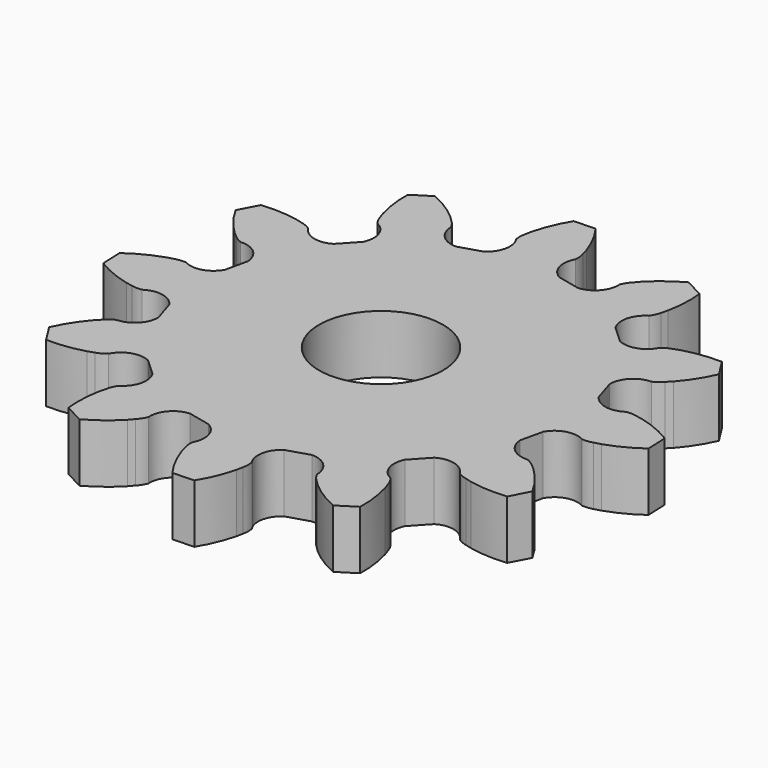
from build123d import *

# Parameters (mm, degrees)
F0_R     = 3.175
F1_DEPTH = 6
F2_R     = 6.35
F3_DEPTH = 6


# Not quite as in the source:
# - ends of sketch curves that miss each other by under 0.0002 mm in the source are joined


with BuildPart() as f1:
    # F0 (on Top) → F1 (new body)
    with BuildSketch(Plane.XY):
        with BuildLine():
            ThreePointArc((8.0856551802, 20.4586539905), (7.495744634, 18.7245439088), (5.8524138883, 17.9154726581))
            Line((5.8524138883, 17.9154726581), (3.533593868, 18.4377149703))
            ThreePointArc((3.533593868, 18.4377149703), (2.39577008, 19.8731553984), (2.6062168473, 21.6927279818))
            ThreePointArc((2.6062168473, 21.6927279818), (2.5956181006, 22.2379348343), (2.4812105153, 22.7711081757))
            Line((2.4812105153, 22.7711081757), (2.304819868, 23.4221699703))
            ThreePointArc((2.304819868, 23.4221699703), (1.5537928627, 25.1976657599), (0.5382999658, 26.8363240419))
            Line((0.5382999658, 26.8363240419), (-1.652266132, 26.7480479703))
            ThreePointArc((-1.652266132, 26.7480479703), (-2.5326105159, 25.0329912972), (-3.1383352523, 23.202821))
            Line((-3.1383352523, 23.202821), (-3.261765132, 22.5396759703))
            ThreePointArc((-3.261765132, 22.5396759703), (-3.3328999602, 21.9990293129), (-3.299595445, 21.4547409207))
            ThreePointArc((-3.299595445, 21.4547409207), (-2.9434159043, 19.6579951944), (-3.962046635, 18.1356532254))
            Line((-3.962046635, 18.1356532254), (-6.231325132, 17.4285189703))
            ThreePointArc((-6.231325132, 17.4285189703), (-7.9344291384, 18.1027349909), (-8.6619631428, 19.7837539701))
            ThreePointArc((-8.6619631428, 19.7837539701), (-8.9437456025, 20.2506173173), (-9.3094119635, 20.6551551548))
            Line((-9.3094119635, 20.6551551548), (-9.787702132, 21.1307969703))
            ThreePointArc((-9.787702132, 21.1307969703), (-11.3258583806, 22.2929078915), (-13.0246300842, 23.2042810788))
            Line((-13.0246300842, 23.2042810788), (-14.877578132, 22.0325489703))
            ThreePointArc((-14.877578132, 22.0325489703), (-14.7824500692, 20.1070937471), (-14.3919378876, 18.2192570409))
            Line((-14.3919378876, 18.2192570409), (-14.167259132, 17.5832419703))
            ThreePointArc((-14.167259132, 17.5832419703), (-13.9585396302, 17.0794612267), (-13.6575531356, 16.6247459674))
            ThreePointArc((-13.6575531356, 16.6247459674), (-12.450720223, 15.2468077423), (-12.5717095188, 13.4191061613))
            Line((-12.5717095188, 13.4191061613), (-14.183394132, 11.6720709703))
            ThreePointArc((-14.183394132, 11.6720709703), (-15.9954339265, 11.4044064302), (-17.4660067474, 12.4964452005))
            ThreePointArc((-17.4660067474, 12.4964452005), (-17.9434693275, 12.7598688849), (-18.4624142066, 12.9273756305))
            Line((-18.4624142066, 12.9273756305), (-19.114446132, 13.1001489703))
            ThreePointArc((-19.114446132, 13.1001489703), (-21.0275840666, 13.3374876551), (-22.954450043, 13.2773741537))
            Line((-22.954450043, 13.2773741537), (-23.973284132, 11.3361509703))
            ThreePointArc((-23.973284132, 11.3361509703), (-22.9281735093, 9.7162222135), (-21.646062089, 8.276564015))
            Line((-21.646062089, 8.276564015), (-21.133476132, 7.8380979703))
            ThreePointArc((-21.133476132, 7.8380979703), (-20.700829784, 7.5061704221), (-20.2128101981, 7.2628687982))
            ThreePointArc((-20.2128101981, 7.2628687982), (-18.4786930704, 6.6729557362), (-17.6696218198, 5.0296249905))
            Line((-17.6696218198, 5.0296249905), (-18.191865132, 2.7108049703))
            ThreePointArc((-18.191865132, 2.7108049703), (-19.6273047939, 1.5729811157), (-21.4468771435, 1.7834279496))
            ThreePointArc((-21.4468771435, 1.7834279496), (-21.992083996, 1.7728292029), (-22.5252573374, 1.6584216176))
            Line((-22.5252573374, 1.6584216176), (-23.176320132, 1.4820309703))
            ThreePointArc((-23.176320132, 1.4820309703), (-24.951815701, 0.7310035617), (-26.5904738545, -0.2844894086))
            Line((-26.5904738545, -0.2844894086), (-26.502198132, -2.4750550297))
            ThreePointArc((-26.502198132, -2.4750550297), (-24.7871404994, -3.3553983967), (-22.9569699288, -3.9611232076))
            Line((-22.9569699288, -3.9611232076), (-22.293825132, -4.0845540297))
            ThreePointArc((-22.293825132, -4.0845540297), (-21.7531784746, -4.1556888579), (-21.2088900824, -4.1223843427))
            ThreePointArc((-21.2088900824, -4.1223843427), (-19.4121448118, -3.7662049106), (-17.8898035408, -4.7848353025))
            Line((-17.8898035408, -4.7848353025), (-17.182669132, -7.0541130297))
            ThreePointArc((-17.182669132, -7.0541130297), (-17.8568848047, -8.7572176771), (-19.5379041318, -9.4847520406))
            ThreePointArc((-19.5379041318, -9.4847520406), (-20.0047679489, -9.7665338494), (-20.4093058145, -10.1322004067))
            Line((-20.4093058145, -10.1322004067), (-20.884947132, -10.6104910297))
            ThreePointArc((-20.884947132, -10.6104910297), (-22.0470577895, -12.1486474277), (-22.9584307722, -13.8474191883))
            Line((-22.9584307722, -13.8474191883), (-21.786699132, -15.7003670297))
            ThreePointArc((-21.786699132, -15.7003670297), (-19.8612438949, -15.6052379651), (-17.9734072026, -15.2147257853))
            Line((-17.9734072026, -15.2147257853), (-17.337391132, -14.9900470297))
            ThreePointArc((-17.337391132, -14.9900470297), (-16.8336102162, -14.7813279046), (-16.3788950361, -14.4803411482))
            ThreePointArc((-16.3788950361, -14.4803411482), (-15.0009577532, -13.2735084084), (-13.1732557298, -13.3944972155))
            Line((-13.1732557298, -13.3944972155), (-11.426220132, -15.0061830297))
            ThreePointArc((-11.426220132, -15.0061830297), (-11.1585555293, -16.8182225752), (-12.2505939215, -18.2887953813))
            ThreePointArc((-12.2505939215, -18.2887953813), (-12.5140190857, -18.7662573158), (-12.6815259557, -19.2852028487))
            Line((-12.6815259557, -19.2852028487), (-12.854298132, -19.9372350297))
            ThreePointArc((-12.854298132, -19.9372350297), (-13.0916378147, -21.8503729188), (-13.0315243037, -23.7772390484))
            Line((-13.0315243037, -23.7772390484), (-11.090300132, -24.7960730297))
            ThreePointArc((-11.090300132, -24.7960730297), (-9.4703714624, -23.7509617127), (-8.0307131966, -22.4688499676))
            Line((-8.0307131966, -22.4688499676), (-7.592247132, -21.9562650297))
            ThreePointArc((-7.592247132, -21.9562650297), (-7.2603195838, -21.5236186817), (-7.0170179599, -21.0355990958))
            ThreePointArc((-7.0170179599, -21.0355990958), (-6.4271048979, -19.3014819682), (-4.7837741522, -18.4924107175))
            Line((-4.7837741522, -18.4924107175), (-2.464955132, -19.0146530297))
            ThreePointArc((-2.464955132, -19.0146530297), (-1.3271304637, -20.4500930376), (-1.5375771112, -22.2696660413))
            ThreePointArc((-1.5375771112, -22.2696660413), (-1.526978382, -22.8148727434), (-1.4125708708, -23.3480459468))
            Line((-1.4125708708, -23.3480459468), (-1.236180132, -23.9991090297))
            ThreePointArc((-1.236180132, -23.9991090297), (-0.4851536505, -25.7746047396), (0.5303392469, -27.4132627523))
            Line((0.5303392469, -27.4132627523), (2.720904868, -27.3249870297))
            ThreePointArc((2.720904868, -27.3249870297), (3.6012490873, -25.6099297494), (4.2069739883, -23.7797590594))
            Line((4.2069739883, -23.7797590594), (4.330403868, -23.1166140297))
            ThreePointArc((4.330403868, -23.1166140297), (4.4015386962, -22.5759673723), (4.368234181, -22.0316789801))
            ThreePointArc((4.368234181, -22.0316789801), (4.012054776, -20.2349335738), (5.0306858327, -18.7125919768))
            Line((5.0306858327, -18.7125919768), (7.299963868, -18.0054580297))
            ThreePointArc((7.299963868, -18.0054580297), (9.003068504, -18.6796726914), (9.7306028786, -20.3606920138))
            ThreePointArc((9.7306028786, -20.3606920138), (10.0123843385, -20.8275553767), (10.3780506996, -21.2320932142))
            Line((10.3780506996, -21.2320932142), (10.856340868, -21.7077350297))
            ThreePointArc((10.856340868, -21.7077350297), (12.3944972864, -22.8698460597), (14.0932691892, -23.7812193009))
            Line((14.0932691892, -23.7812193009), (15.946216868, -22.6094870297))
            ThreePointArc((15.946216868, -22.6094870297), (15.8510888659, -20.684032283), (15.4605768903, -18.7961960233))
            Line((15.4605768903, -18.7961960233), (15.235897868, -18.1601800297))
            ThreePointArc((15.235897868, -18.1601800297), (15.0271791498, -17.6563988792), (14.7261924755, -17.2016835377))
            ThreePointArc((14.7261924755, -17.2016835377), (13.5193592467, -15.8237466509), (13.6403480539, -13.9960446276))
            Line((13.6403480539, -13.9960446276), (15.252033868, -12.2490090297))
            ThreePointArc((15.252033868, -12.2490090297), (17.0640734135, -11.981344427), (18.5346462196, -13.0733828192))
            ThreePointArc((18.5346462196, -13.0733828192), (19.0121081541, -13.3368079834), (19.531053687, -13.5043148535))
            Line((19.531053687, -13.5043148535), (20.183085868, -13.6770870297))
            ThreePointArc((20.183085868, -13.6770870297), (22.0962237431, -13.9144267579), (24.023089875, -13.8543130938))
            Line((24.023089875, -13.8543130938), (25.041923868, -11.9130890297))
            ThreePointArc((25.041923868, -11.9130890297), (23.9968119132, -10.2931608362), (22.7147003254, -8.8535025939))
            Line((22.7147003254, -8.8535025939), (22.202114868, -8.4150360297))
            ThreePointArc((22.202114868, -8.4150360297), (21.76946852, -8.0831084815), (21.2814489341, -7.8398068576))
            ThreePointArc((21.2814489341, -7.8398068576), (19.5473327821, -7.2498937743), (18.7382615517, -5.6065629853))
            Line((18.7382615517, -5.6065629853), (19.260503868, -3.2877430297))
            ThreePointArc((19.260503868, -3.2877430297), (20.6959438759, -2.1499193614), (22.515516116, -2.360365584))
            ThreePointArc((22.515516116, -2.360365584), (23.0607226131, -2.349767392), (23.5938958766, -2.2353600569))
            Line((23.5938958766, -2.2353600569), (24.244958868, -2.0589690297))
            ThreePointArc((24.244958868, -2.0589690297), (26.0204546576, -1.3079420244), (27.6591129397, -0.2924491275))
            Line((27.6591129397, -0.2924491275), (27.570836868, 1.8981169703))
            ThreePointArc((27.570836868, 1.8981169703), (25.8557796831, 2.7784601496), (24.0256096072, 3.3841849152))
            Line((24.0256096072, 3.3841849152), (23.362464868, 3.5076159703))
            ThreePointArc((23.362464868, 3.5076159703), (22.8218180787, 3.5787497682), (22.277529794, 3.5454454378))
            ThreePointArc((22.277529794, 3.5454454378), (20.4807842278, 3.1892667155), (18.9584425848, 4.2078967813))
            Line((18.9584425848, 4.2078967813), (18.251307868, 6.4771749703))
            ThreePointArc((18.251307868, 6.4771749703), (18.9255235407, 8.1802796176), (20.6065428678, 8.9078139811))
            ThreePointArc((20.6065428678, 8.9078139811), (21.0734066849, 9.18959579), (21.4779445505, 9.5552623473))
            Line((21.4779445505, 9.5552623473), (21.953585868, 10.0335529703))
            ThreePointArc((21.953585868, 10.0335529703), (23.115697238, 11.5717089195), (24.0270703456, 13.2704807598))
            Line((24.0270703456, 13.2704807598), (22.855337868, 15.1234279703))
            ThreePointArc((22.855337868, 15.1234279703), (20.9298826448, 15.0282999075), (19.0420459386, 14.6377877259))
            Line((19.0420459386, 14.6377877259), (18.406030868, 14.4131089703))
            ThreePointArc((18.406030868, 14.4131089703), (17.9022497175, 14.2043902521), (17.447534376, 13.9034035778))
            ThreePointArc((17.447534376, 13.9034035778), (16.0695968549, 12.6965701341), (14.241894662, 12.8175595532))
            Line((14.241894662, 12.8175595532), (12.494859868, 14.4292449703))
            ThreePointArc((12.494859868, 14.4292449703), (12.2271952653, 16.2412845157), (13.3192336575, 17.7118573219))
            ThreePointArc((13.3192336575, 17.7118573219), (13.5826579764, 18.189319614), (13.7501647378, 18.7082649989))
            Line((13.7501647378, 18.7082649989), (13.922937868, 19.3602969703))
            ThreePointArc((13.922937868, 19.3602969703), (14.1602765983, 21.2734348909), (14.1001629438, 23.2003008696))
            Line((14.1001629438, 23.2003008696), (12.158939868, 24.2191349703))
            ThreePointArc((12.158939868, 24.2191349703), (10.5390105485, 23.1740239196), (9.0993519326, 21.8919119082))
            Line((9.0993519326, 21.8919119082), (8.660885868, 21.3793269703))
            ThreePointArc((8.660885868, 21.3793269703), (8.3289580725, 20.9466802264), (8.0856551802, 20.4586539905))
        make_face()
        with Locations((0.535841868, -0.2906590297)):
            Circle(F0_R, mode=Mode.SUBTRACT)
    extrude(amount=F1_DEPTH)

    # F2 (on Top) → F3 (cut)
    with BuildSketch(Plane.XY):
        Circle(F2_R)
    extrude(amount=F3_DEPTH, mode=Mode.SUBTRACT)


solid = f1.part
